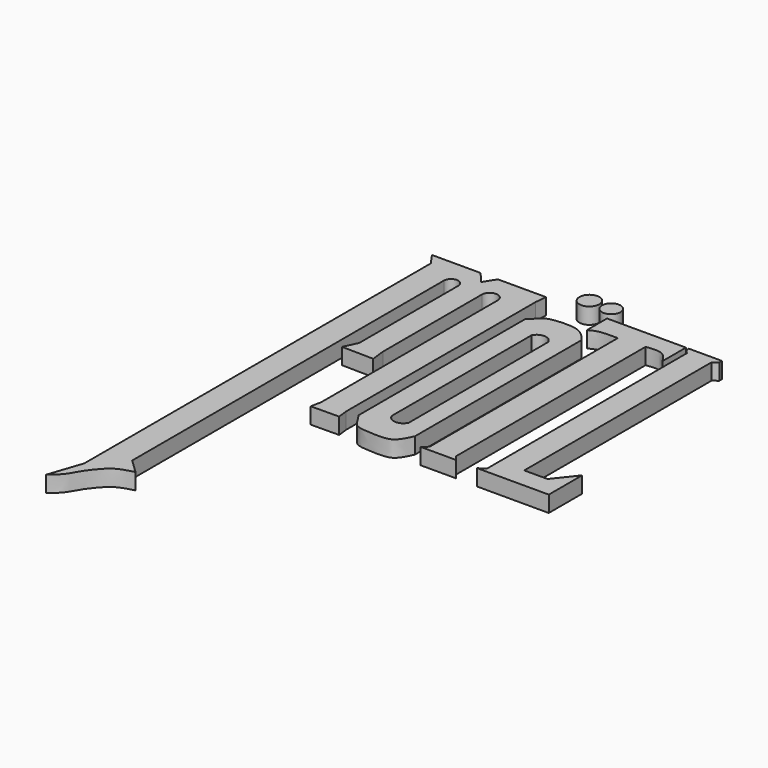
from build123d import *

# Parameters (mm, degrees)
F1_DEPTH = 2
F0_R     = 1.2293027529
F0_R_2   = 1.1387722668


with BuildPart() as f1:
    # F0 (on Top) → F1 (new body)
    with BuildSketch(Plane.XY):
        with BuildLine():
            Line((-56.4536973834, -6.1546978541), (-57.8551329672, -10.3112254292))
            add(Edge.make_bspline(
                [(-57.8551329672, -10.3112254292), (-57.3990056054, -9.9414517987), (-56.4859601505, -9.1536799978), (-55.9236162382, -7.9625439336), (-55.3275550964, -7.0871377477), (-54.5572435837, -6.1064735999), (-53.5728500895, -5.1965475686), (-52.8687499464, -4.8594879918), (-51.4612309635, -4.492750857)],
                knots=[0, 0, 0, 0, 0.1851248852, 0.3424784316, 0.4841918055, 0.6386525718, 0.7854964076, 1, 1, 1, 1], degree=3))
            Line((-51.4612309635, -4.492750857), (-53.2226637006, -2.8122463264))
            Line((-53.2226637006, -2.8122463264), (-53.2226637006, 45.3190617263))
            ThreePointArc((-53.2226637006, 45.3190617263), (-52.341947332, 46.1997780949), (-51.4612309635, 45.3190617263))
            Line((-51.4612309635, 45.3190617263), (-51.4612309635, 30.0551969558))
            Line((-51.4612309635, 30.0551969558), (-52.242167294, 28.371186927))
            Line((-52.242167294, 28.371186927), (-48.3424975936, 28.3045752825))
            Line((-48.3424975936, 28.3045752825), (-48.5432296991, 30.0551969558))
            Line((-48.5432296991, 30.0551969558), (-48.5432296991, 45.3190617263))
            ThreePointArc((-48.5432296991, 45.3190617263), (-47.5677810609, 46.2945103645), (-46.5923324227, 45.3190617263))
            Line((-46.5923324227, 45.3190617263), (-46.5923324227, 18.1011855602))
            Line((-46.5923324227, 18.1011855602), (-46.84920609, 16.7881511152))
            Line((-46.84920609, 16.7881511152), (-43.3698035777, 16.8244559318))
            Line((-43.3698035777, 16.8244559318), (-43.5161976447, 18.1011855602))
            Line((-43.5161976447, 18.1011855602), (-43.5161976447, 47.3245307803))
            Line((-43.5161976447, 47.3245307803), (-43.3698035777, 48.7729273736))
            Line((-43.3698035777, 48.7729273736), (-49.3231341243, 48.7729273736))
            Line((-49.3231341243, 48.7729273736), (-50.2144545317, 47.3245307803))
            Line((-50.2144545317, 47.3245307803), (-51.4612309635, 48.7729273736))
            Line((-51.4612309635, 48.7729273736), (-57.456433773, 48.7729273736))
            Line((-57.456433773, 48.7729273736), (-56.4536973834, 47.3245307803))
            Line((-56.4536973834, 47.3245307803), (-56.4536973834, -6.1546978541))
        make_face()
    extrude(amount=F1_DEPTH)


with BuildPart() as f1b:
    # F0 (on Top) → F1, piece 2 (new body)
    with BuildSketch(Plane.XY):
        with BuildLine():
            add(Edge.make_bspline(
                [(-42.0775525272, 43.8902974129), (-41.6942788959, 44.2154963908), (-41.036405557, 45.1327555061), (-39.8109964401, 45.5680290153), (-37.2395787485, 45.6733438975), (-35.9250489528, 44.9708525517), (-35.3615108781, 44.240565625), (-35.0915975869, 43.8902974129)],
                knots=[0, 0, 0, 0, 0.1971875376, 0.3772673806, 0.6274257288, 0.8183607775, 1, 1, 1, 1], degree=3))
            Line((-42.0775525272, 43.8902974129), (-42.0775525272, 18.1802082807))
            add(Edge.make_bspline(
                [(-42.0775525272, 18.1802082807), (-41.9429261615, 18.0153509456), (-41.6240175614, 17.6248299533), (-41.0127698726, 16.2664561335), (-39.2658081646, 16.0518243935), (-36.7606634204, 15.992326804), (-36.0911249212, 16.5025921155), (-35.642160255, 17.0346677821), (-35.2946967023, 17.757625575), (-35.0915975869, 18.1802082807)],
                knots=[0, 0, 0, 0, 0.1090973313, 0.258434349, 0.429378141, 0.6341982103, 0.7471561555, 0.8522079201, 1, 1, 1, 1], degree=3))
            Line((-35.0915975869, 18.1802082807), (-35.0915975869, 43.8902974129))
        make_face()
        with BuildLine():
            ThreePointArc((-39.486374706, 41.6832044721), (-38.3841825965, 42.3262593723), (-37.3506359756, 41.5778420866))
            Line((-37.3506359756, 41.5778420866), (-37.3176857829, 19.9997238815))
            ThreePointArc((-37.3176857829, 19.9997238815), (-38.4506574535, 19.3340583356), (-39.5020097494, 20.1223436743))
            Line((-39.5020097494, 20.1223436743), (-39.486374706, 41.6832044721))
        make_face(mode=Mode.SUBTRACT)
    extrude(amount=F1_DEPTH)


with BuildPart() as f1c:
    # F0 (on Top) → F1, piece 3 (new body)
    with BuildSketch(Plane.XY):
        with Locations((-39.6497291513, 50.8133545518)):
            Circle(F0_R)
    extrude(amount=F1_DEPTH)


with BuildPart() as f1d:
    # F0 (on Top) → F1, piece 4 (new body)
    with BuildSketch(Plane.XY):
        with Locations((-36.9417816401, 50.8029596414)):
            Circle(F0_R_2)
    extrude(amount=F1_DEPTH)


with BuildPart() as f1e:
    # F0 (on Top) → F1, piece 5 (new body)
    with BuildSketch(Plane.XY):
        with BuildLine():
            add(Edge.make_bspline(
                [(-35.9943732619, 45.8593294024), (-35.9943732619, 46.8966551125), (-35.9943732619, 47.9339808226), (-35.9943732619, 48.9713065326)],
                knots=[0, 0, 0, 0, 3.1119771302, 3.1119771302, 3.1119771302, 3.1119771302], degree=3))
            add(Edge.make_bspline(
                [(-35.9943732619, 45.8593294024), (-35.6848569517, 46.0290729346), (-34.9317656783, 46.4420798379), (-33.4773216876, 46.4231020734), (-32.6206460595, 46.4119240642)],
                knots=[0, 0, 0, 0, 0.4109944188, 1, 1, 1, 1], degree=3))
            Line((-32.6206460595, 46.4119240642), (-32.6206460595, 17.3571370542))
            Line((-32.6206460595, 17.3571370542), (-33.2751534879, 16.7897772044))
            Line((-33.2751534879, 16.7897772044), (-28.9125721902, 16.7897772044))
            Line((-28.9125721902, 16.7897772044), (-29.3923355639, 17.4005385488))
            Line((-29.3923355639, 17.4005385488), (-29.3923355639, 46.6736778617))
            add(Edge.make_bspline(
                [(-26.251276955, 45.3649051487), (-26.5624442676, 45.8622749418), (-27.2196972414, 46.9128280121), (-28.642918623, 46.7561688922), (-29.3923355639, 46.6736778617)],
                knots=[0, 0, 0, 0, 0.4734361425, 1, 1, 1, 1], degree=3))
            Line((-26.251276955, 45.3649051487), (-26.251276955, 48.9713065326))
            add(Edge.make_bspline(
                [(-35.9943732619, 48.9713065326), (-32.746674493, 48.9713065326), (-29.498975724, 48.9713065326), (-26.251276955, 48.9713065326)],
                knots=[0, 0, 0, 0, 9.7430963069, 9.7430963069, 9.7430963069, 9.7430963069], degree=3))
        make_face()
    extrude(amount=F1_DEPTH)


with BuildPart() as f1f:
    # F0 (on Top) → F1, piece 6 (new body)
    with BuildSketch(Plane.XY):
        Polygon((-25.8890558034, 48.5697090626), (-25.4468992352, 48.1069870293), (-25.4468992352, 17.2156337649), (-26.251276955, 16.7265031487), (-17.3976588994, 16.7265031487), (-17.3976588994, 21.8868292868), (-19.5253770798, 19.1966127604), (-22.4032197148, 19.1966127604), (-22.4032197148, 48.1069870293), (-21.8068230897, 48.5697090626), (-21.8068230897, 48.9713065326), (-25.8890558034, 48.9713065326), align=None)
    extrude(amount=F1_DEPTH)


solid = Compound([f1.part, f1b.part, f1c.part, f1d.part, f1e.part, f1f.part])
